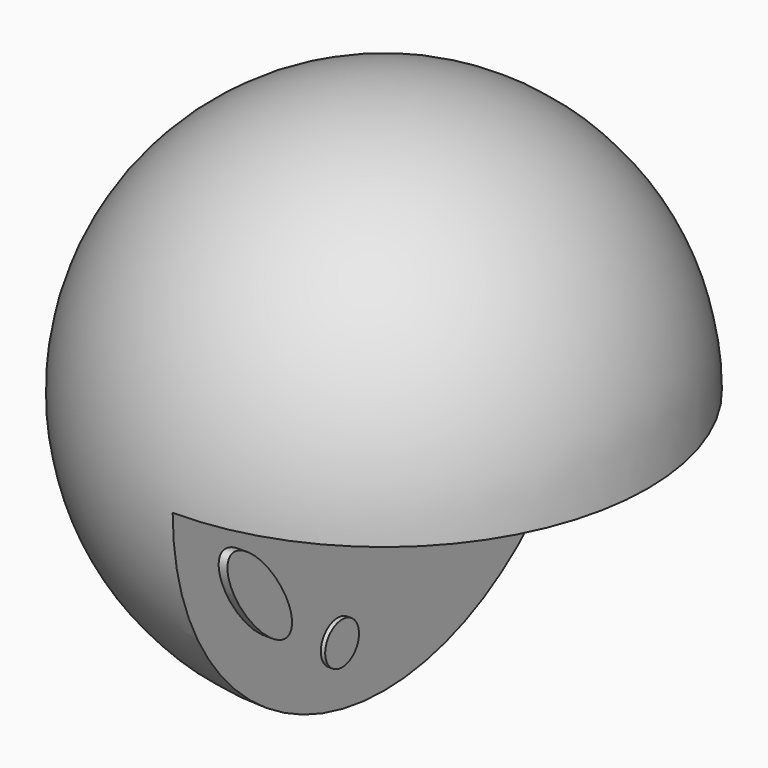
from build123d import *

# Parameters (mm, degrees)
F1_ANGLE  = 270
F5_DEPTH  = 1
F7_DEPTH  = 1
F8_R      = 2.3999784267
F9_DEPTH  = 0.5
F10_R     = 2.2479266401
F11_DEPTH = 0.5
F12_R     = 2.219715214
F13_DEPTH = 0.5
F14_R     = 2.225517588
F15_DEPTH = 0.5
F21_DEPTH = 1


# Not quite as in the source:
# - the program builds the solid bodies; features that only make, move or delete a surface that nothing else refers to are left out


with BuildPart() as f1:
    # F0 (on Right) → F1 (revolve)
    with BuildSketch(Plane.YZ):
        with BuildLine():
            Line((30.0334315861, 0), (-29.9665684139, 0))
            ThreePointArc((-29.9665684139, 0), (0.0334315861, -30), (30.0334315861, 0))
        make_face()
    revolve(axis=Axis((0, 0.0334315861, 0), (0, 1, 0)), revolution_arc=F1_ANGLE)

    # F2 (on face) → F3 (revolve)
    with BuildSketch(Plane.YZ):
        with BuildLine():
            Line((0, -13.9990693861), (0, 0))
            Line((0, 0), (-0.1614197102, 0))
            ThreePointArc((-0.1614197102, 0), (-7.0802445482, -7.0802445482), (0, -13.9990693861))
        make_face()
        with BuildLine():
            Line((0, -13.9990693861), (0, 0))
            ThreePointArc((0, 0), (-7.0807098551, -6.9995346931), (0, -13.9990693861))
        make_face()
    revolve(axis=Axis((0, 0, -6.9995346931), (0, 0, -1)))

    # F4 (on Right) → F5 (join)
    with BuildSketch(Plane.YZ):
        with BuildLine():
            add(Edge.make_bspline(
                [(17.0095134526, -15.6440958381), (20.8283990638, -15.6440958381), (18.9189562582, -6.4476504922), (17.0095134526, 2.7487948537), (15.1000706471, -6.4476504922), (13.1906278415, -15.6440958381), (17.0095134526, -15.6440958381)],
                knots=[0, 0, 0, 2.0943951024, 2.0943951024, 4.1887902048, 4.1887902048, 6.2831853072, 6.2831853072, 6.2831853072], degree=2, weights=[1, 0.5, 1, 0.5, 1, 0.5, 1]))
        make_face()
    extrude(amount=F5_DEPTH)

    # F6 (on Right) → F7 (join)
    with BuildSketch(Plane.YZ):
        with BuildLine():
            add(Edge.make_bspline(
                [(-14.6672427654, -18.0654972792), (-11.4328069704, -15.6641534543), (-19.325768114, -8.4118548322), (-27.2187292576, -1.15955621), (-22.560203909, -10.8131986571), (-17.9016785604, -20.4668411041), (-14.6672427654, -18.0654972792)],
                knots=[0, 0, 0, 2.0943951024, 2.0943951024, 4.1887902048, 4.1887902048, 6.2831853072, 6.2831853072, 6.2831853072], degree=2, weights=[1, 0.5, 1, 0.5, 1, 0.5, 1]))
        make_face()
    extrude(amount=F7_DEPTH)

    # F8 (on face) → F9 (join)
    with BuildSketch(Plane.YZ):
        with Locations((-6.5264105797, -22.420451045)):
            Circle(F8_R)
    extrude(amount=F9_DEPTH)

    # F10 (on face) → F11 (join)
    with BuildSketch(Plane(origin=(0, 0, 0), x_dir=(1, 0, 0), z_dir=(0, 0, -1))):
        with Locations((5.2993446589, -22.5904844701)):
            Circle(F10_R)
    extrude(amount=F11_DEPTH)

    # F12 (on face) → F13 (join)
    with BuildSketch(Plane(origin=(0, 0, 0), x_dir=(1, 0, 0), z_dir=(0, 0, -1))):
        with Locations((25.2750441432, 3.729365766)):
            Circle(F12_R)
    extrude(amount=F13_DEPTH)

    # F14 (on face) → F15 (join)
    with BuildSketch(Plane(origin=(0, 0, 0), x_dir=(1, 0, 0), z_dir=(0, 0, -1))):
        with Locations((11.6383302957, 21.1235657334)):
            Circle(F14_R)
    extrude(amount=F15_DEPTH)

    # F20 (on face) → F21 (join)
    with BuildSketch(Plane(origin=(0, 0, 0), x_dir=(1, 0, 0), z_dir=(0, 0, -1))):
        with BuildLine():
            add(Edge.make_bspline(
                [(7.3144584894, -10.2911405265), (10.5177671604, -12.9900925853), (13.6132754829, -6.0656891234), (16.7087838054, 0.8587143384), (10.4099668119, -3.3667370647), (4.1111498184, -7.5921884678), (7.3144584894, -10.2911405265)],
                knots=[0, 0, 0, 2.0943951024, 2.0943951024, 4.1887902048, 4.1887902048, 6.2831853072, 6.2831853072, 6.2831853072], degree=2, weights=[1, 0.5, 1, 0.5, 1, 0.5, 1]))
        make_face()
    extrude(amount=F21_DEPTH)


solid = f1.part
